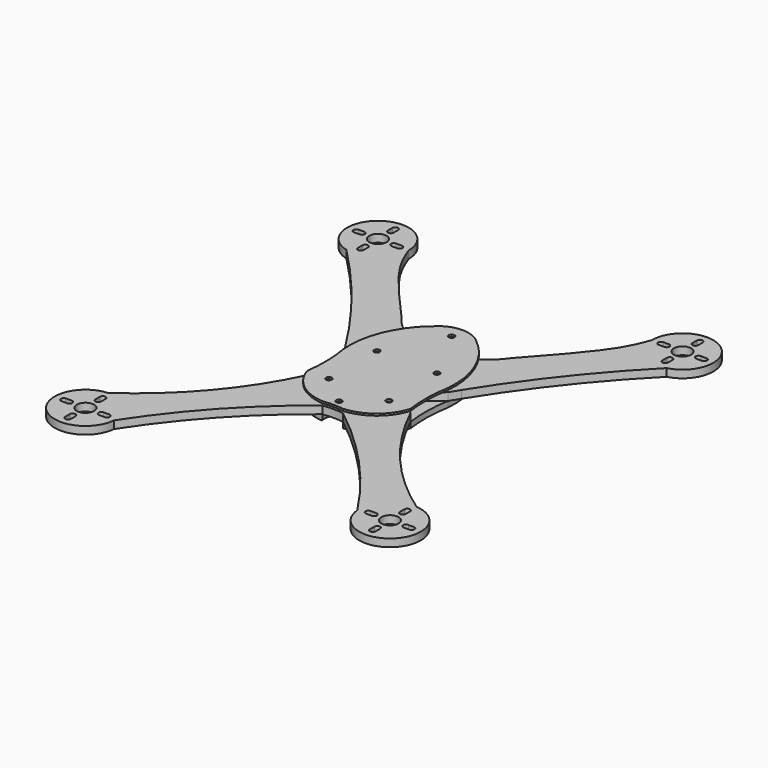
from build123d import *

# Parameters (mm, degrees)
F2_R     = 4.5
F2_R_2   = 1.5
F3_DEPTH = 4
F4_DEPTH = 3
F2_R_3   = 4.5172540556
F7_DEPTH = 6
F8_DEPTH = 5


# Not quite as in the source:
# - a feature of the source that left no trace in its solid (it failed there, or was rolled back) is left out


with BuildPart() as f3:
    # F2 (on Top) → F3 (new body)
    with BuildSketch(Plane.XY):
        with BuildLine():
            ThreePointArc((-83.2531983557, 98.3113630516), (-54.8830214905, 66.2093397503), (-30.222153937, 31.1772338056))
            ThreePointArc((-30.222153937, 31.1772338056), (-35.4158370921, 46.8554181645), (-35.0131206214, 63.3665546775))
            ThreePointArc((-35.0131206214, 63.3665546775), (-32.268330545, 65.9408130686), (-28.5100138802, 65.7517768946))
            add(Edge.make_bspline(
                [(-28.5100138802, 65.7517768946), (-39.5508731031, 78.058687756), (-57.2145769654, 97.7478826388), (-61.5768803406, 109.4043854936), (-63.2124861993, 113.7748849114)],
                knots=[0, 0, 0, 0, 0.6250591217, 1, 1, 1, 1], degree=3))
            ThreePointArc((-63.2124861994, 113.7748849114), (-88.986735794, 126.4601575764), (-83.2531983557, 98.3113630516))
        make_face()
        with BuildLine():
            Line((-90.4521688223, 115.2927249074), (-87.5107913613, 115.2927249074))
            ThreePointArc((-87.5107913613, 115.2927249074), (-86.4501311896, 114.8533850792), (-86.0107913613, 113.7927249074))
            ThreePointArc((-86.0107913613, 113.7927249074), (-86.4501311896, 112.7320647356), (-87.5107913613, 112.2927249074))
            Line((-87.5107913613, 112.2927249074), (-90.4521688223, 112.2927249074))
            ThreePointArc((-90.4521688223, 112.2927249074), (-91.9521688223, 113.7927249074), (-90.4521688223, 115.2927249074))
        make_face(mode=Mode.SUBTRACT)
        with BuildLine():
            Line((-80.7124762535, 102.5519296527), (-80.7124762535, 105.4933071136))
            ThreePointArc((-80.7124762535, 105.4933071136), (-79.2124762535, 106.9933071136), (-77.7124762535, 105.4933071136))
            Line((-77.7124762535, 105.4933071136), (-77.7124762535, 102.5519296527))
            ThreePointArc((-77.7124762535, 102.5519296527), (-79.2124762535, 101.0519296527), (-80.7124762535, 102.5519296527))
        make_face(mode=Mode.SUBTRACT)
        with Locations((-79.2124762535, 113.7927249074)):
            Circle(F2_R, mode=Mode.SUBTRACT)
        with BuildLine():
            ThreePointArc((-77.7124762535, 122.0921427011), (-79.2124762535, 120.5921427011), (-80.7124762535, 122.0921427011))
            Line((-80.7124762535, 122.0921427011), (-80.7124762535, 125.0335201621))
            ThreePointArc((-80.7124762535, 125.0335201621), (-79.2124762535, 126.5335201621), (-77.7124762535, 125.0335201621))
            Line((-77.7124762535, 125.0335201621), (-77.7124762535, 122.0921427011))
        make_face(mode=Mode.SUBTRACT)
        with BuildLine():
            ThreePointArc((-70.9119557738, 112.2927249074), (-72.4119557738, 113.7927249074), (-70.9119557738, 115.2927249074))
            Line((-70.9119557738, 115.2927249074), (-67.9705783129, 115.2927249074))
            ThreePointArc((-67.9705783129, 115.2927249074), (-66.4705783129, 113.7927249074), (-67.9705783129, 112.2927249074))
            Line((-67.9705783129, 112.2927249074), (-70.9119557738, 112.2927249074))
        make_face(mode=Mode.SUBTRACT)
        with BuildLine():
            ThreePointArc((-27.2539428433, 26.3454403678), (0, 15.1357500676), (27.2539428433, 26.3454403678))
            ThreePointArc((27.2539428433, 26.3454403678), (25.8313338836, 42.1816963864), (19.0153788674, 56.5467086786))
            ThreePointArc((19.0153788674, 56.5467086786), (0, 50.8868121764), (-19.0153788674, 56.5467086786))
            ThreePointArc((-19.0153788674, 56.5467086786), (-25.8313338836, 42.1816963864), (-27.2539428433, 26.3454403678))
        make_face()
        with BuildLine():
            ThreePointArc((-17.1132667707, 33.6132667707), (-15.6132667707, 35.1132667707), (-14.1132667707, 33.6132667707))
            ThreePointArc((-14.1132667707, 33.6132667707), (-15.6132667707, 32.1132667707), (-17.1132667707, 33.6132667707))
        make_face(mode=Mode.SUBTRACT)
        with Locations((15.6132667707, 33.6132667707)):
            Circle(F2_R_2, mode=Mode.SUBTRACT)
        with BuildLine():
            ThreePointArc((35.0131206214, 63.3665546775), (35.4158370921, 46.8554181646), (30.2221539371, 31.1772338058))
            ThreePointArc((30.2221539371, 31.1772338058), (54.8830214905, 66.2093397504), (83.2531983557, 98.3113630516))
            ThreePointArc((83.2531983557, 98.3113630516), (88.986735794, 126.4601575764), (63.2124861993, 113.7748849114))
            add(Edge.make_bspline(
                [(28.5100138802, 65.7517768946), (39.5508731031, 78.058687756), (57.2145769654, 97.7478826388), (61.5768803406, 109.4043854936), (63.2124861993, 113.7748849114)],
                knots=[0, 0, 0, 0, 0.6250591217, 1, 1, 1, 1], degree=3))
            ThreePointArc((28.5100138802, 65.7517768946), (32.268330545, 65.9408130686), (35.0131206214, 63.3665546775))
        make_face()
        with BuildLine():
            ThreePointArc((70.9119557738, 115.2927249074), (72.4119557738, 113.7927249074), (70.9119557738, 112.2927249074))
            Line((70.9119557738, 112.2927249074), (67.9705783129, 112.2927249074))
            ThreePointArc((67.9705783129, 112.2927249074), (66.4705783129, 113.7927249074), (67.9705783129, 115.2927249074))
            Line((67.9705783129, 115.2927249074), (70.9119557738, 115.2927249074))
        make_face(mode=Mode.SUBTRACT)
        with BuildLine():
            Line((77.7124762535, 102.5519296527), (77.7124762535, 105.4933071136))
            ThreePointArc((77.7124762535, 105.4933071136), (79.2124762535, 106.9933071136), (80.7124762535, 105.4933071136))
            Line((80.7124762535, 105.4933071136), (80.7124762535, 102.5519296527))
            ThreePointArc((80.7124762535, 102.5519296527), (79.2124762535, 101.0519296527), (77.7124762535, 102.5519296527))
        make_face(mode=Mode.SUBTRACT)
        with Locations((79.2124762535, 113.7927249074)):
            Circle(F2_R, mode=Mode.SUBTRACT)
        with BuildLine():
            Line((90.4521688223, 112.2927249074), (87.5107913613, 112.2927249074))
            ThreePointArc((87.5107913613, 112.2927249074), (86.4501311896, 112.7320647356), (86.0107913613, 113.7927249074))
            ThreePointArc((86.0107913613, 113.7927249074), (86.4501311896, 114.8533850792), (87.5107913613, 115.2927249074))
            Line((87.5107913613, 115.2927249074), (90.4521688223, 115.2927249074))
            ThreePointArc((90.4521688223, 115.2927249074), (91.9521688223, 113.7927249074), (90.4521688223, 112.2927249074))
        make_face(mode=Mode.SUBTRACT)
        with BuildLine():
            ThreePointArc((77.7124762535, 125.0335201621), (79.2124762535, 126.5335201621), (80.7124762535, 125.0335201621))
            Line((80.7124762535, 125.0335201621), (80.7124762535, 122.0921427011))
            ThreePointArc((80.7124762535, 122.0921427011), (79.2124762535, 120.5921427011), (77.7124762535, 122.0921427011))
            Line((77.7124762535, 122.0921427011), (77.7124762535, 125.0335201621))
        make_face(mode=Mode.SUBTRACT)
        with BuildLine():
            ThreePointArc((-30.222153937, 31.1772338056), (-28.729227545, 28.7667558056), (-27.2539428433, 26.3454403678))
            ThreePointArc((-27.2539428433, 26.3454403678), (-25.8313338836, 42.1816963864), (-19.0153788674, 56.5467086786))
            ThreePointArc((-19.0153788674, 56.5467086786), (-24.2043190189, 60.6937278757), (-28.5100138802, 65.7517768946))
            ThreePointArc((-28.5100138802, 65.7517768946), (-32.268330545, 65.9408130686), (-35.0131206214, 63.3665546775))
            ThreePointArc((-35.0131206214, 63.3665546775), (-35.4158370921, 46.8554181645), (-30.222153937, 31.1772338056))
        make_face()
        with BuildLine():
            ThreePointArc((19.0153788674, 56.5467086786), (25.8313338836, 42.1816963864), (27.2539428433, 26.3454403678))
            ThreePointArc((27.2539428433, 26.3454403678), (28.7292275451, 28.7667558057), (30.2221539371, 31.1772338058))
            ThreePointArc((30.2221539371, 31.1772338058), (35.4158370921, 46.8554181646), (35.0131206214, 63.3665546775))
            ThreePointArc((35.0131206214, 63.3665546775), (32.268330545, 65.9408130686), (28.5100138802, 65.7517768946))
            ThreePointArc((28.5100138802, 65.7517768946), (24.2043190189, 60.6937278757), (19.0153788674, 56.5467086786))
        make_face()
    extrude(amount=F3_DEPTH)


with BuildPart() as f3b:
    # F2 (on Top) → F3, piece 2 (new body)
    with BuildSketch(Plane.XY):
        with BuildLine():
            ThreePointArc((-5.3660199046, -14.6965133653), (-18.7459429949, -9.5157029864), (-26.8234012705, 2.3425349051))
            ThreePointArc((-26.8234012705, 2.3425349051), (-49.4326206455, -32.5844969249), (-80.326573153, -60.4527234861))
            ThreePointArc((-80.326573153, -60.4527234861), (-90.6197958728, -87.6332048228), (-63.2720276132, -77.7930538648))
            ThreePointArc((-63.2720276132, -77.7930538648), (-36.9574280607, -43.8234232896), (-5.3660199046, -14.6965133653))
        make_face()
        with BuildLine():
            Line((-80.7124762535, -87.6546837389), (-80.7124762535, -84.713306278))
            ThreePointArc((-80.7124762535, -84.713306278), (-79.2124762535, -83.213306278), (-77.7124762535, -84.713306278))
            Line((-77.7124762535, -84.713306278), (-77.7124762535, -87.6546837389))
            ThreePointArc((-77.7124762535, -87.6546837389), (-79.2124762535, -89.1546837389), (-80.7124762535, -87.6546837389))
        make_face(mode=Mode.SUBTRACT)
        with BuildLine():
            ThreePointArc((-86.0107913613, -76.4138884842), (-86.4501311896, -77.474548656), (-87.5107913613, -77.9138884842))
            Line((-87.5107913613, -77.9138884842), (-90.4521688223, -77.9138884842))
            ThreePointArc((-90.4521688223, -77.9138884842), (-91.9521688223, -76.4138884842), (-90.4521688223, -74.9138884842))
            Line((-90.4521688223, -74.9138884842), (-87.5107913613, -74.9138884842))
            ThreePointArc((-87.5107913613, -74.9138884842), (-86.4501311896, -75.3532283125), (-86.0107913613, -76.4138884842))
        make_face(mode=Mode.SUBTRACT)
        with Locations((-79.2124762535, -76.4138884842)):
            Circle(F2_R, mode=Mode.SUBTRACT)
        with BuildLine():
            Line((-77.7124762535, -65.1730932295), (-77.7124762535, -68.1144706905))
            ThreePointArc((-77.7124762535, -68.1144706905), (-79.2124762535, -69.6144706905), (-80.7124762535, -68.1144706905))
            Line((-80.7124762535, -68.1144706905), (-80.7124762535, -65.1730932295))
            ThreePointArc((-80.7124762535, -65.1730932295), (-79.2124762535, -63.6730932295), (-77.7124762535, -65.1730932295))
        make_face(mode=Mode.SUBTRACT)
        with BuildLine():
            Line((-67.9705783129, -77.9138884842), (-70.9119557738, -77.9138884842))
            ThreePointArc((-70.9119557738, -77.9138884842), (-72.4119557738, -76.4138884842), (-70.9119557738, -74.9138884842))
            Line((-70.9119557738, -74.9138884842), (-67.9705783129, -74.9138884842))
            ThreePointArc((-67.9705783129, -74.9138884842), (-66.4705783129, -76.4138884842), (-67.9705783129, -77.9138884842))
        make_face(mode=Mode.SUBTRACT)
        with BuildLine():
            ThreePointArc((80.326573153, -60.4527234861), (49.4326206455, -32.5844969249), (26.8234012705, 2.3425349051))
            ThreePointArc((26.8234012705, 2.3425349051), (18.7459429949, -9.5157029864), (5.3660199046, -14.6965133653))
            ThreePointArc((5.3660199046, -14.6965133653), (36.9574280607, -43.8234232896), (63.2720276132, -77.7930538648))
            ThreePointArc((63.2720276132, -77.7930538648), (90.6197958728, -87.6332048227), (80.326573153, -60.4527234861))
        make_face()
        with BuildLine():
            ThreePointArc((70.9119557738, -74.9138884842), (72.4119557738, -76.4138884842), (70.9119557738, -77.9138884842))
            Line((70.9119557738, -77.9138884842), (67.9705783129, -77.9138884842))
            ThreePointArc((67.9705783129, -77.9138884842), (66.4705783129, -76.4138884842), (67.9705783129, -74.9138884842))
            Line((67.9705783129, -74.9138884842), (70.9119557738, -74.9138884842))
        make_face(mode=Mode.SUBTRACT)
        with BuildLine():
            ThreePointArc((77.7124762535, -84.713306278), (79.2124762535, -83.213306278), (80.7124762535, -84.713306278))
            Line((80.7124762535, -84.713306278), (80.7124762535, -87.6546837389))
            ThreePointArc((80.7124762535, -87.6546837389), (79.2124762535, -89.1546837389), (77.7124762535, -87.6546837389))
            Line((77.7124762535, -87.6546837389), (77.7124762535, -84.713306278))
        make_face(mode=Mode.SUBTRACT)
        with Locations((79.2124762535, -76.4138884842)):
            Circle(F2_R, mode=Mode.SUBTRACT)
        with BuildLine():
            ThreePointArc((80.7124762535, -68.1144706905), (79.2124762535, -69.6144706905), (77.7124762535, -68.1144706905))
            Line((77.7124762535, -68.1144706905), (77.7124762535, -65.1730932295))
            ThreePointArc((77.7124762535, -65.1730932295), (79.2124762535, -63.6730932295), (80.7124762535, -65.1730932295))
            Line((80.7124762535, -65.1730932295), (80.7124762535, -68.1144706905))
        make_face(mode=Mode.SUBTRACT)
        with BuildLine():
            ThreePointArc((86.0107913613, -76.4138884842), (86.4501311896, -75.3532283125), (87.5107913613, -74.9138884842))
            Line((87.5107913613, -74.9138884842), (90.4521688223, -74.9138884842))
            ThreePointArc((90.4521688223, -74.9138884842), (91.9521688223, -76.4138884842), (90.4521688223, -77.9138884842))
            Line((90.4521688223, -77.9138884842), (87.5107913613, -77.9138884842))
            ThreePointArc((87.5107913613, -77.9138884842), (86.4501311896, -77.474548656), (86.0107913613, -76.4138884842))
        make_face(mode=Mode.SUBTRACT)
        with BuildLine():
            ThreePointArc((5.3660199046, -14.6965133653), (18.7459429949, -9.5157029864), (26.8234012705, 2.3425349051))
            ThreePointArc((26.8234012705, 2.3425349051), (0, 14.7787581859), (-26.8234012705, 2.3425349051))
            ThreePointArc((-26.8234012705, 2.3425349051), (-18.7459429949, -9.5157029864), (-5.3660199046, -14.6965133653))
            ThreePointArc((-5.3660199046, -14.6965133653), (0, -6.6413932777), (5.3660199046, -14.6965133653))
        make_face()
        with BuildLine():
            ThreePointArc((-17.1132667707, 2.3867332293), (-15.6132667707, 3.8867332293), (-14.1132667707, 2.3867332293))
            ThreePointArc((-14.1132667707, 2.3867332293), (-15.6132667707, 0.8867332293), (-17.1132667707, 2.3867332293))
        make_face(mode=Mode.SUBTRACT)
        with BuildLine():
            ThreePointArc((17.1132667707, 2.3867332293), (15.6132667707, 0.8867332293), (14.1132667707, 2.3867332293))
            ThreePointArc((14.1132667707, 2.3867332293), (15.6132667707, 3.8867332293), (17.1132667707, 2.3867332293))
        make_face(mode=Mode.SUBTRACT)
        with BuildLine():
            ThreePointArc((-5.3660199046, -14.6965133653), (0, -14.3281621986), (5.3660199046, -14.6965133653))
            ThreePointArc((5.3660199046, -14.6965133653), (0, -6.6413932777), (-5.3660199046, -14.6965133653))
        make_face()
        with Locations((0, -10.4859630273)):
            Circle(F2_R_2, mode=Mode.SUBTRACT)
    extrude(amount=F3_DEPTH)


with BuildPart() as f4:
    # F2 (on Top) → F4 (new body)
    with BuildSketch(Plane.XY):
        with BuildLine():
            ThreePointArc((-27.2539428433, 26.3454403678), (0, 15.1357500676), (27.2539428433, 26.3454403678))
            ThreePointArc((27.2539428433, 26.3454403678), (25.8313338836, 42.1816963864), (19.0153788674, 56.5467086786))
            ThreePointArc((19.0153788674, 56.5467086786), (0, 50.8868121764), (-19.0153788674, 56.5467086786))
            ThreePointArc((-19.0153788674, 56.5467086786), (-25.8313338836, 42.1816963864), (-27.2539428433, 26.3454403678))
        make_face()
        with BuildLine():
            ThreePointArc((-17.1132667707, 33.6132667707), (-15.6132667707, 35.1132667707), (-14.1132667707, 33.6132667707))
            ThreePointArc((-14.1132667707, 33.6132667707), (-15.6132667707, 32.1132667707), (-17.1132667707, 33.6132667707))
        make_face(mode=Mode.SUBTRACT)
        with Locations((15.6132667707, 33.6132667707)):
            Circle(F2_R_2, mode=Mode.SUBTRACT)
        with BuildLine():
            ThreePointArc((-26.8234012705, 2.3425349051), (0, 14.7787581859), (26.8234012705, 2.3425349051))
            ThreePointArc((26.8234012705, 2.3425349051), (26.0769774848, 14.3612376104), (27.2539428433, 26.3454403678))
            ThreePointArc((27.2539428433, 26.3454403678), (0, 15.1357500676), (-27.2539428433, 26.3454403678))
            ThreePointArc((-27.2539428433, 26.3454403678), (-26.0769774848, 14.3612376104), (-26.8234012705, 2.3425349051))
        make_face()
        with BuildLine():
            ThreePointArc((5.3660199046, -14.6965133653), (18.7459429949, -9.5157029864), (26.8234012705, 2.3425349051))
            ThreePointArc((26.8234012705, 2.3425349051), (0, 14.7787581859), (-26.8234012705, 2.3425349051))
            ThreePointArc((-26.8234012705, 2.3425349051), (-18.7459429949, -9.5157029864), (-5.3660199046, -14.6965133653))
            ThreePointArc((-5.3660199046, -14.6965133653), (0, -6.6413932777), (5.3660199046, -14.6965133653))
        make_face()
        with BuildLine():
            ThreePointArc((-17.1132667707, 2.3867332293), (-15.6132667707, 3.8867332293), (-14.1132667707, 2.3867332293))
            ThreePointArc((-14.1132667707, 2.3867332293), (-15.6132667707, 0.8867332293), (-17.1132667707, 2.3867332293))
        make_face(mode=Mode.SUBTRACT)
        with BuildLine():
            ThreePointArc((17.1132667707, 2.3867332293), (15.6132667707, 0.8867332293), (14.1132667707, 2.3867332293))
            ThreePointArc((14.1132667707, 2.3867332293), (15.6132667707, 3.8867332293), (17.1132667707, 2.3867332293))
        make_face(mode=Mode.SUBTRACT)
    extrude(amount=-F4_DEPTH)


with BuildPart() as f5_1:
    # F5: copy of F4
    add(f4.part.moved(Location((0, 0, 7))))


with BuildPart() as f7:
    # F2 (on Top) → F7 (new body)
    with BuildSketch(Plane.XY):
        with BuildLine():
            ThreePointArc((-19.0153788674, 56.5467086786), (0, 50.8868121764), (19.0153788674, 56.5467086786))
            ThreePointArc((19.0153788674, 56.5467086786), (16.1107989808, 60.2024683457), (12.8447489214, 63.5392452443))
            ThreePointArc((12.8447489214, 63.5392452443), (11.8869686776, 64.2902382765), (11.0133644239, 65.137675081))
            ThreePointArc((11.0133644239, 65.137675081), (0, 69.6982653616), (-11.0133644239, 65.137675081))
            ThreePointArc((-11.0133644239, 65.137675081), (-11.8869686776, 64.2902382765), (-12.8447489214, 63.5392452443))
            ThreePointArc((-12.8447489214, 63.5392452443), (-16.1107989808, 60.2024683457), (-19.0153788674, 56.5467086786))
        make_face()
        with Locations((0.0254183764, 62.7011399201)):
            Circle(F2_R_3, mode=Mode.SUBTRACT)
        with Locations((0.0254183764, 62.7011399201)):
            Circle(F2_R_3)
        with Locations((0.0254183764, 62.7011399201)):
            Circle(F2_R_2, mode=Mode.SUBTRACT)
        with BuildLine():
            ThreePointArc((-27.2539428433, 26.3454403678), (0, 15.1357500676), (27.2539428433, 26.3454403678))
            ThreePointArc((27.2539428433, 26.3454403678), (25.8313338836, 42.1816963864), (19.0153788674, 56.5467086786))
            ThreePointArc((19.0153788674, 56.5467086786), (0, 50.8868121764), (-19.0153788674, 56.5467086786))
            ThreePointArc((-19.0153788674, 56.5467086786), (-25.8313338836, 42.1816963864), (-27.2539428433, 26.3454403678))
        make_face()
        with BuildLine():
            ThreePointArc((-17.1132667707, 33.6132667707), (-15.6132667707, 35.1132667707), (-14.1132667707, 33.6132667707))
            ThreePointArc((-14.1132667707, 33.6132667707), (-15.6132667707, 32.1132667707), (-17.1132667707, 33.6132667707))
        make_face(mode=Mode.SUBTRACT)
        with Locations((15.6132667707, 33.6132667707)):
            Circle(F2_R_2, mode=Mode.SUBTRACT)
        with BuildLine():
            ThreePointArc((-26.8234012705, 2.3425349051), (0, 14.7787581859), (26.8234012705, 2.3425349051))
            ThreePointArc((26.8234012705, 2.3425349051), (26.0769774848, 14.3612376104), (27.2539428433, 26.3454403678))
            ThreePointArc((27.2539428433, 26.3454403678), (0, 15.1357500676), (-27.2539428433, 26.3454403678))
            ThreePointArc((-27.2539428433, 26.3454403678), (-26.0769774848, 14.3612376104), (-26.8234012705, 2.3425349051))
        make_face()
        with BuildLine():
            ThreePointArc((5.3660199046, -14.6965133653), (18.7459429949, -9.5157029864), (26.8234012705, 2.3425349051))
            ThreePointArc((26.8234012705, 2.3425349051), (0, 14.7787581859), (-26.8234012705, 2.3425349051))
            ThreePointArc((-26.8234012705, 2.3425349051), (-18.7459429949, -9.5157029864), (-5.3660199046, -14.6965133653))
            ThreePointArc((-5.3660199046, -14.6965133653), (0, -6.6413932777), (5.3660199046, -14.6965133653))
        make_face()
        with BuildLine():
            ThreePointArc((-17.1132667707, 2.3867332293), (-15.6132667707, 3.8867332293), (-14.1132667707, 2.3867332293))
            ThreePointArc((-14.1132667707, 2.3867332293), (-15.6132667707, 0.8867332293), (-17.1132667707, 2.3867332293))
        make_face(mode=Mode.SUBTRACT)
        with BuildLine():
            ThreePointArc((17.1132667707, 2.3867332293), (15.6132667707, 0.8867332293), (14.1132667707, 2.3867332293))
            ThreePointArc((14.1132667707, 2.3867332293), (15.6132667707, 3.8867332293), (17.1132667707, 2.3867332293))
        make_face(mode=Mode.SUBTRACT)
        with BuildLine():
            ThreePointArc((-5.3660199046, -14.6965133653), (0, -14.3281621986), (5.3660199046, -14.6965133653))
            ThreePointArc((5.3660199046, -14.6965133653), (0, -6.6413932777), (-5.3660199046, -14.6965133653))
        make_face()
        with Locations((0, -10.4859630273)):
            Circle(F2_R_2, mode=Mode.SUBTRACT)
    extrude(amount=F7_DEPTH)

    # F8 (cut): a face of the model
    f8_faces = [f7.faces().sort_by_distance(p)[0] for p in [
        (-4.75691e-05, 25.411619654, 0),
    ]]
    extrude(f8_faces, amount=-F8_DEPTH, mode=Mode.SUBTRACT)


solid = Compound([f3.part, f3b.part, f4.part, f7.part])
